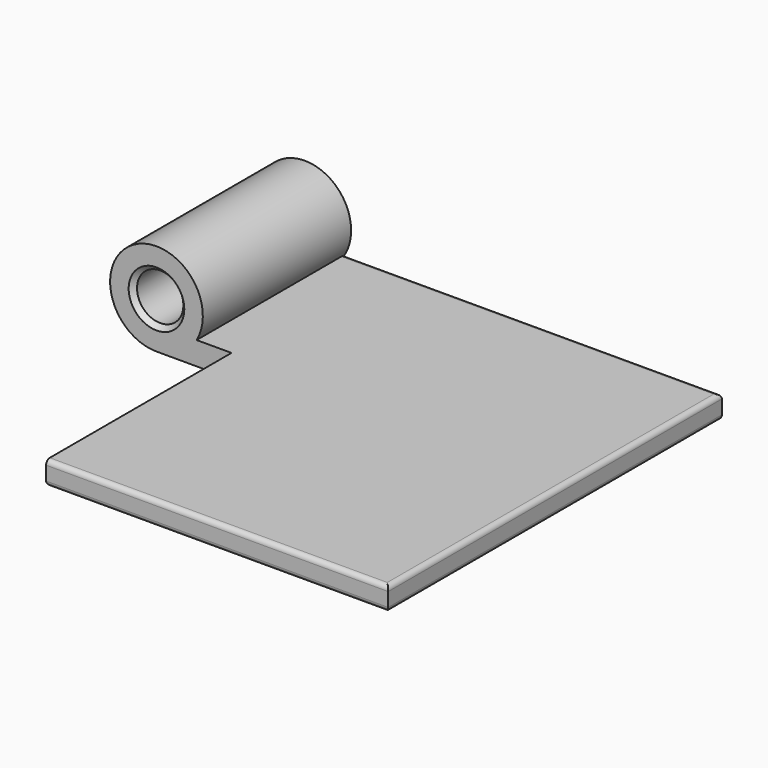
from build123d import *

# Parameters (mm, degrees)
F0_R     = 3.175
F1_DEPTH = 25.4
F0_W     = 46.875538686
F0_H     = 3.175
F2_DEPTH = 57.15
F3_R     = 0.635
F4_SIZE  = 0.635


with BuildPart() as f1:
    # F0 (on Front) → F1 (new body)
    with BuildSketch(Plane.XZ):
        with BuildLine():
            ThreePointArc((5.499261314, -3.175), (-3.175, 5.499261314), (0, -6.35))
            Line((0, -6.35), (10.274461314, -6.35))
            Line((10.274461314, -6.35), (10.274461314, -3.175))
            Line((10.274461314, -3.175), (5.499261314, -3.175))
        make_face()
        Circle(F0_R, mode=Mode.SUBTRACT)
    extrude(amount=F1_DEPTH)

    # F0 (on Front) → F2 (join)
    with BuildSketch(Plane.XZ):
        with Locations((33.712230657, -4.7625)):
            Rectangle(F0_W, F0_H)
    extrude(amount=F2_DEPTH)

    # F3
    f3_edges = [f1.edges().sort_by_distance(p)[0] for p in [
        (33.712231, -57.15, -3.175),
        (33.712231, -57.15, -6.35),
        (57.15, -28.575, -3.175),
        (57.15, -28.575, -6.35),
        (31.324631, 0, -3.175),
        (10.274461, -41.275, -6.35),
    ]]
    fillet(f3_edges, radius=F3_R)

    # F4
    f4_edges = [f1.edges().sort_by_distance(p)[0] for p in [
        (-3.175, -25.4, 0),
        (-3.175, 0, 0),
    ]]
    chamfer(f4_edges, length=F4_SIZE)


solid = f1.part
